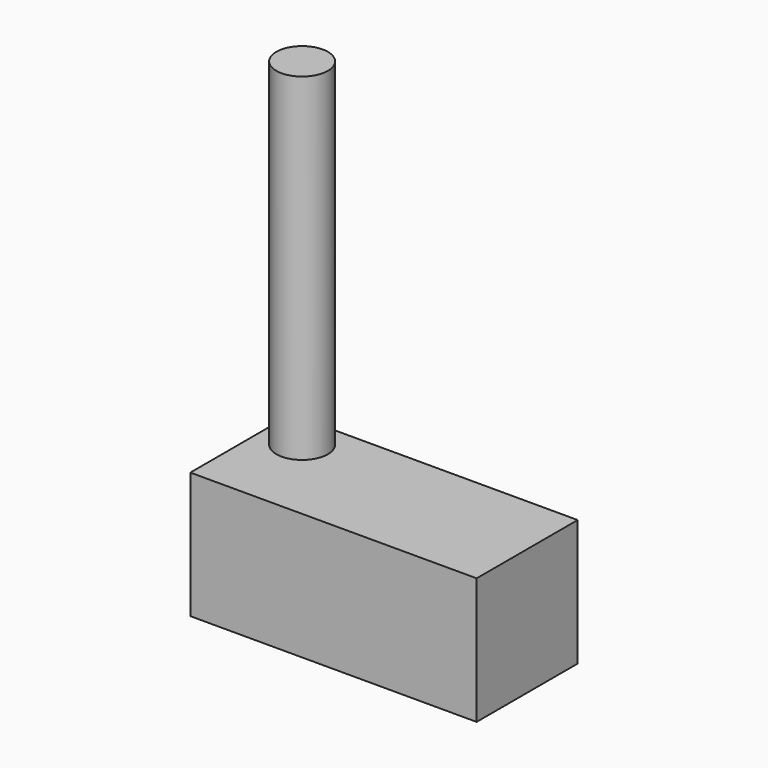
from build123d import *

# Parameters (mm, degrees)
F0_W     = 57.5268156826
F0_H     = 25.3720888868
F1_DEPTH = 25.4
F2_R     = 5.1788015889
F3_DEPTH = 67.8203047


# Not quite as in the source:
# - an extrude ends at something that could not be found from the text; its depth is read off the source's solid


with BuildPart() as f1:
    # F0 (on Top) → F1 (new body)
    with BuildSketch(Plane.XY):
        with Locations((-0.1256037503, 4.5217587613)):
            Rectangle(F0_W, F0_H)
    extrude(amount=F1_DEPTH)

    # F2 (on face) → F3 (join, through all)
    with BuildSketch(Plane.XY.offset(25.4)):
        with Locations((-21.1015380919, 10.1739559323)):
            Circle(F2_R)
    extrude(amount=F3_DEPTH)


solid = f1.part
